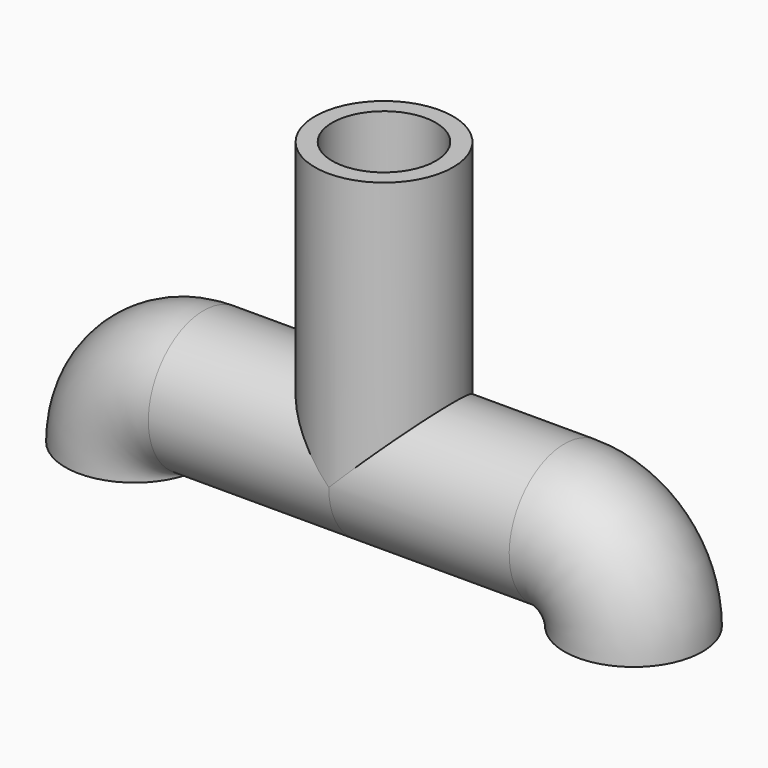
from build123d import *
from build123d import SkipClean  # not in build123d's __all__

# Parameters (mm, degrees)
F0_R      = 1
F0_R_2    = 0.75
F4_DEPTH  = 2.61254
F5_DEPTH  = 2.61254
F8_R      = 1
F8_R_2    = 0.75
F9_DEPTH  = 4
F10_R     = 0.75
F11_DEPTH = 4
F13_R     = 0.75
F14_DEPTH = 4


# Not quite as in the source:
# - after a boolean that leaves OpenCascade's solid faulty, fix() repairs it


with BuildPart() as f2:
    # F2: sweep along a path in F1
    with BuildLine(Plane.XZ) as f2_path:
        ThreePointArc((-2.61254, 1), (-3.3196467812, 0.7071067812), (-3.61254, 0))
    # F0 (on Top) → F2 (sweep)
    with BuildSketch(Plane.XY):
        with Locations((-3.61254, 0)):
            Circle(F0_R)
        with Locations((-3.61254, 0)):
            Circle(F0_R_2, mode=Mode.SUBTRACT)
    sweep(path=f2_path.line)

    # F5 (add): a face of the model
    f5_faces = [f2.faces().sort_by_distance(p)[0] for p in [
        (-2.61254, 0, 1.9717157288),
    ]]


with BuildPart() as f3:
    # F3: sweep along a path in F1
    with BuildLine(Plane.XZ) as f3_path:
        ThreePointArc((2.61254, 1), (3.3196467812, 0.7071067812), (3.61254, 0))
    # F0 (on Top) → F3 (sweep)
    with BuildSketch(Plane.XY):
        with BuildLine():
            ThreePointArc((4.61254, 0), (3.61254, 1), (2.61254, 0))
            ThreePointArc((2.61254, 0), (3.61254, -1), (4.61254, 0))
        make_face()
        with BuildLine():
            ThreePointArc((4.36254, 0), (3.61254, -0.75), (2.86254, 0))
            ThreePointArc((2.86254, 0), (3.61254, 0.75), (4.36254, 0))
        make_face(mode=Mode.SUBTRACT)
    sweep(path=f3_path.line)

    # F4 (add): a face of the model
    f4_faces = [f3.faces().sort_by_distance(p)[0] for p in [
        (2.61254, 0.9717157288, 1),
    ]]
    extrude(f4_faces, amount=F4_DEPTH)


with BuildPart() as f2_1:
    add(f2.part, clean=False)

    add(f3.part)  # F5 merges F3
    extrude(f5_faces, amount=F5_DEPTH)

    # F6: union 

    # F8 (on offset) → F9 (join)
    with BuildSketch(Plane.XY.offset(1)):
        Circle(F8_R)
        Circle(F8_R_2, mode=Mode.SUBTRACT)
    with SkipClean():  # cleaning this boolean's faces spoils the solid; the shape is the same uncleaned
        extrude(amount=F9_DEPTH)

    # F10 (on face) → F11 (cut)
    with BuildSketch(Plane.XY.offset(5)):
        Circle(F10_R)
    extrude(amount=-F11_DEPTH, mode=Mode.SUBTRACT)

    add(f2_1.part.fix(), mode=Mode.REPLACE)

    # F13 (on offset) → F14 (cut)
    with BuildSketch(Plane.YZ.offset(2)):
        with Locations((0, 1)):
            Circle(F13_R)
    extrude(amount=-F14_DEPTH, mode=Mode.SUBTRACT)


solid = f2_1.part
